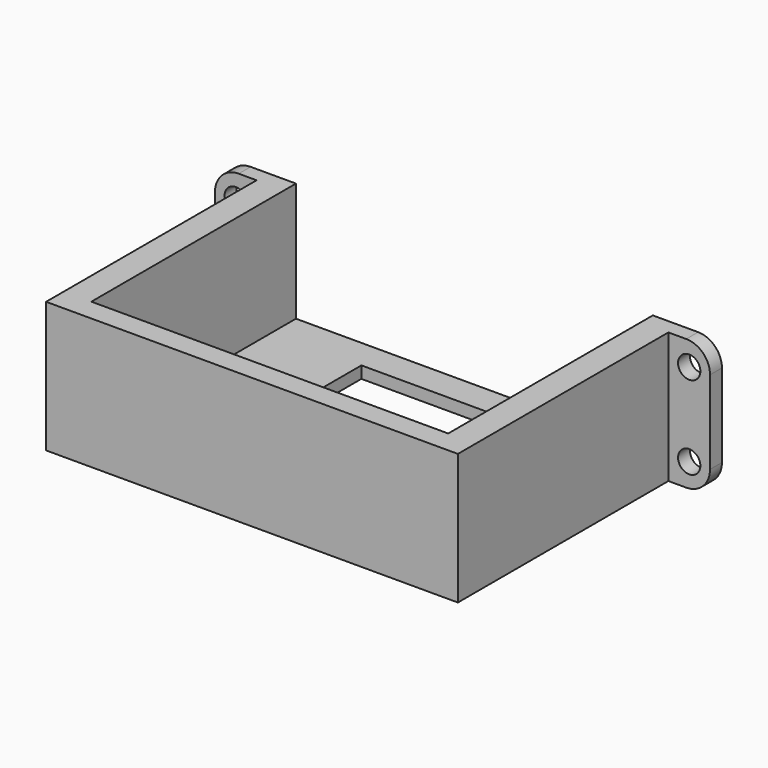
from build123d import *

# Parameters (mm, degrees)
F1_DEPTH  = 25.4
F2_W      = 87.9329293966
F2_H      = 59.3619965534
F3_DEPTH  = 2.54
F4_W      = 8.89
F4_H      = 27.94
F5_DEPTH  = 3.175
F7_DEPTH  = 2.541
F8_R      = 5.08
F9_R      = 2.38125
F10_DEPTH = 3.176


# Not quite as in the source:
# - a feature names something its author has since deleted; it is built from what else it names


with BuildPart() as f1:
    # F0 (on Top) → F1 (new body)
    with BuildSketch(Plane.XY):
        Polygon((38.1, -54.61), (-38.1, -54.61), (-38.1, 0), (-43.9664646983, 0), (-43.9664646983, -59.3619965534), (43.9664646983, -59.3619965534), (43.9664646983, 0), (38.1, 0), align=None)
    extrude(amount=F1_DEPTH)

    # F2 (on face) → F3 (join)
    with BuildSketch(Plane(origin=(0, 0, 0), x_dir=(1, 0, 0), z_dir=(0, 0, -1))):
        with Locations((0, 29.6809982767)):
            Rectangle(F2_W, F2_H)
    extrude(amount=F3_DEPTH)

    # F4 (on face) → F5 (join)
    with BuildSketch(Plane(origin=(0, 0, 0), x_dir=(-1, 0, 0), z_dir=(0, 1, 0))):
        with Locations((-48.4114646983, 11.43)):
            Rectangle(F4_W, F4_H)
        with Locations((48.4114646983, 11.43)):
            Rectangle(F4_W, F4_H)
    extrude(amount=-F5_DEPTH)

    # F6 (on face) → F7 (cut, through all)
    with BuildSketch(Plane.XY):
        Polygon((0, -6.35), (-19.05, -6.35), (-19.05, -41.91), (0, -41.91), (19.05, -41.91), (19.05, -6.35), align=None)
    extrude(amount=-F7_DEPTH, mode=Mode.SUBTRACT)

    # F8
    f8_edges = [f1.edges().sort_by_distance(p)[0] for p in [
        (52.856465, -1.5875, 25.4),
        (-52.856465, -1.5875, 25.4),
        (-52.856465, -1.5875, -2.54),
        (52.856465, -1.5875, -2.54),
    ]]
    fillet(f8_edges, radius=F8_R)

    # F9 (on face) → F10 (cut, through all)
    with BuildSketch(Plane.XZ.offset(3.175)):
        with Locations((48.4114646983, 20.32)):
            Circle(F9_R)
        with Locations((48.4114646983, 2.54)):
            Circle(F9_R)
        with Locations((-48.4114646983, 2.54)):
            Circle(F9_R)
        with Locations((-48.4114646983, 20.32)):
            Circle(F9_R)
    extrude(amount=-F10_DEPTH, mode=Mode.SUBTRACT)


solid = f1.part
